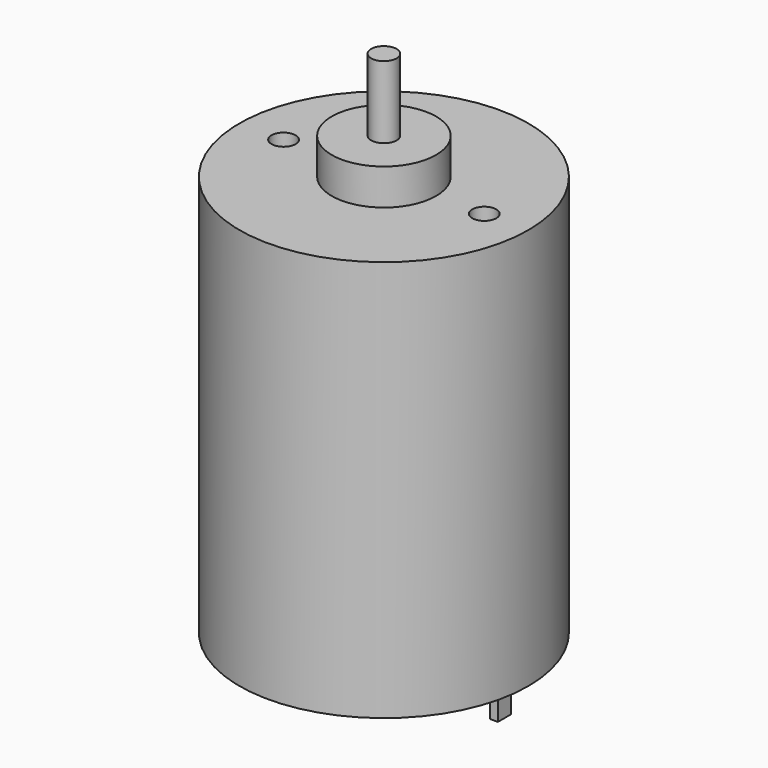
from build123d import *

# Parameters (mm, degrees)
F0_R      = 18
F1_DEPTH  = 25
F2_R      = 6.5
F3_DEPTH  = 4.5
F4_R      = 1.5875
F5_DEPTH  = 9
F6_W      = 1
F6_H      = 2
F7_DEPTH  = 4.5
F8_R      = 1.5
F9_DEPTH  = 5
F10_R     = 2.5
F11_DEPTH = 4.5


# Not quite as in the source:
# - a pattern or mirror of a feature is missing from the dataset's text; its kind, count and spacing are read off the source's solid


with BuildPart() as f1:
    # F0 (on Top) → F1 (new body, symmetric)
    with BuildSketch(Plane.XY):
        Circle(F0_R)
    extrude(amount=F1_DEPTH, both=True)

    # F2 (on face) → F3 (join)
    with BuildSketch(Plane.XY.offset(25)):
        Circle(F2_R)
    extrude(amount=F3_DEPTH)

    # F4 (on face) → F5 (join)
    with BuildSketch(Plane.XY.offset(29.5)):
        Circle(F4_R)
    extrude(amount=F5_DEPTH)

    # F6 (on face) → F7 (join)
    with BuildSketch(Plane(origin=(0, 0, -25), x_dir=(1, 0, 0), z_dir=(0, 0, -1))):
        with Locations((-14.5, 0)):
            Rectangle(F6_W, F6_H)
    f7 = extrude(amount=F7_DEPTH)

    # F7_copies: F7 across plane
    add(f7.mirror(Plane(origin=(0, 0, 0), x_dir=(0, 0, 1), z_dir=(1, 0, 0))))

    # F8 (on face) → F9 (cut)
    with BuildSketch(Plane.XY.offset(25)):
        with Locations((12.5, 0)):
            Circle(F8_R)
        with Locations((-12.5, 0)):
            Circle(F8_R)
    extrude(amount=-F9_DEPTH, mode=Mode.SUBTRACT)

    # F10 (on face) → F11 (join)
    with BuildSketch(Plane(origin=(0, 0, -25), x_dir=(1, 0, 0), z_dir=(0, 0, -1))):
        Circle(F10_R)
    extrude(amount=F11_DEPTH)


solid = f1.part
